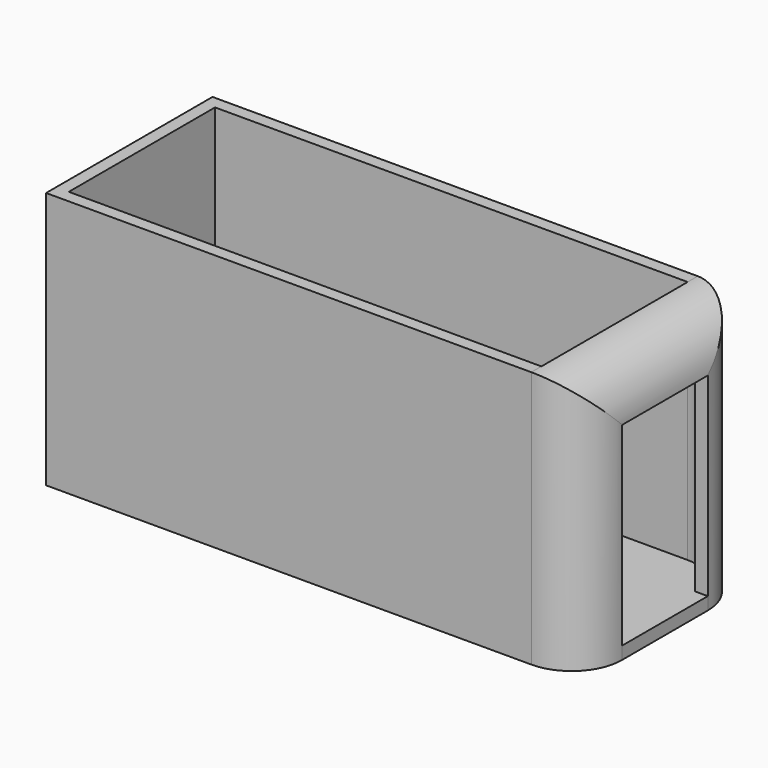
from build123d import *

# Parameters (mm, degrees)
F0_W     = 106.154050678
F0_H     = 41.2226635963
F1_DEPTH = 51
F2_R     = 10
F3_T     = -2.5


# Not quite as in the source:
# - a shell that OpenCascade refuses in one call is made with other operations: the cavity is built on its own and cut out


with BuildPart() as f1:
    # F0 (on Top) → F1 (new body)
    with BuildSketch(Plane.XY):
        with Locations((2.456812188, -44.6538021788)):
            Rectangle(F0_W, F0_H)
    extrude(amount=F1_DEPTH)

    # F2
    f2_edges = [f1.edges().sort_by_distance(p)[0] for p in [
        (55.533838, -65.265134, 25.5),
        (55.533838, -24.04247, 25.5),
        (55.533838, -44.653802, 51),
    ]]
    fillet(f2_edges, radius=F2_R)

    # F3: a shell. OpenCascade refuses it in one call, so the cavity is built on its own and cut out:
    # the body offset inwards by the wall thickness, plus a prism from it out through each open face.
    f3_core = offset(f1.part, amount=F3_T, mode=Mode.PRIVATE)
    f3_exits = [f3_core.faces().sort_by_distance(p)[0] for p in [
        (-1.293188, -44.653802, 48.5),
        (53.033838, -44.653802, 21.75),
    ]]
    add(f3_core, mode=Mode.SUBTRACT)
    extrude(f3_exits, amount=-F3_T, mode=Mode.SUBTRACT)


solid = f1.part
